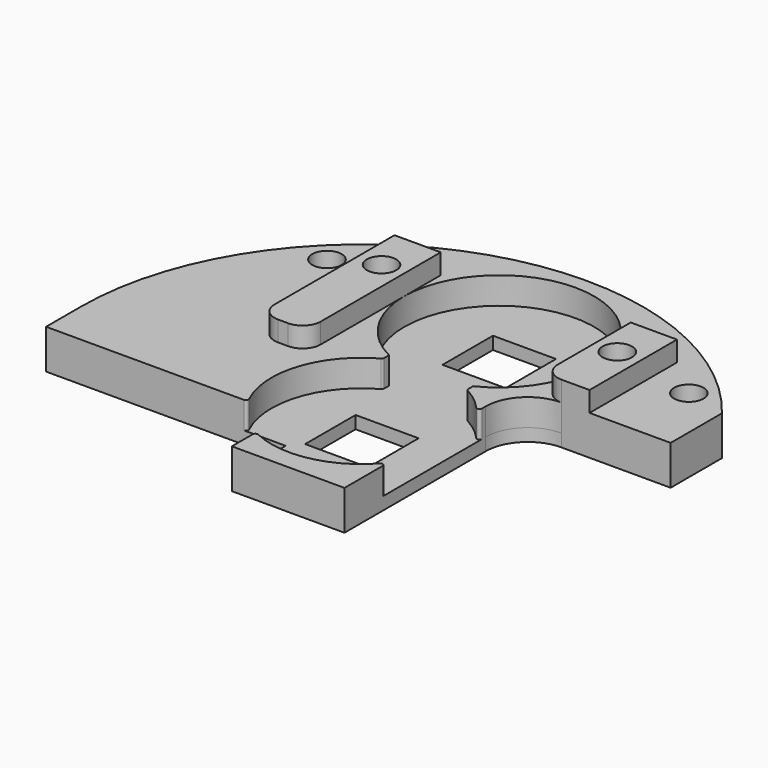
from build123d import *

# Parameters (mm, degrees)
F0_W      = 66.9
F0_H      = 51.6
F1_DEPTH  = 1.5
F2_R      = 33.44999
F3_R      = 1.75
F5_DEPTH  = 10
F6_W      = 60
F6_H      = 1.5
F7_DEPTH  = 7
F8_W      = 28.5
F8_H      = 1.5
F9_DEPTH  = 13
F10_W     = 18
F10_H     = 1.5
F11_DEPTH = 31
F12_R     = 5
F13_R     = 1.75
F13_R_2   = 11.3
F15_DEPTH = 3.2
F16_R     = 10.7
F17_DEPTH = 3.2
F18_W     = 10
F18_H     = 8
F19_DEPTH = 5
F14_W     = 7.5
F14_H     = 7.5
F20_DEPTH = 25
F21_W     = 13.4
F21_H     = 4.7
F22_DEPTH = 5
F23_W     = 5.5
F23_H     = 20
F23_H_2   = 13
F24_DEPTH = 2.4
F25_R     = 1.75
F26_DEPTH = 25
F27_R     = 2.15
F28_R     = 0.3


# Not quite as in the source:
# - a fillet or chamfer is up to 0.001 mm smaller than in the source, because OpenCascade refuses the exact size
# - ends of sketch curves that miss each other by under 0.0002 mm in the source are joined


with BuildPart() as f1:
    # F0 (on Top) → F1 (new body)
    with BuildSketch(Plane.XY):
        Rectangle(F0_W, F0_H)
    extrude(amount=F1_DEPTH)

    # F2 (radius 33.45 in the source; OpenCascade refuses exactly that, so slightly less here)
    f2_edges = [f1.edges().sort_by_distance(p)[0] for p in [
        (-33.45, 25.8, 0.75),
        (33.45, 25.8, 0.75),
    ]]
    fillet(f2_edges, radius=F2_R)

    # F3 (on Top) → F5 (cut)
    with BuildSketch(Plane.XY):
        with Locations((-21.525, 14.0641658831)):
            Circle(F3_R)
        with Locations((-14.025, 12.8033463032)):
            Circle(F3_R)
        with Locations((21.525, 14.0641658831)):
            Circle(F3_R)
        with Locations((14.025, 12.8033463032)):
            Circle(F3_R)
    extrude(amount=F5_DEPTH, mode=Mode.SUBTRACT)

    # F6 (on face) → F7 (cut)
    with BuildSketch(Plane.YZ.offset(33.45)):
        with Locations((4.2, 0.75)):
            Rectangle(F6_W, F6_H)
    extrude(amount=-F7_DEPTH, mode=Mode.SUBTRACT)

    # F8 (on face) → F9 (cut)
    with BuildSketch(Plane.XZ.offset(25.8)):
        with Locations((-19.2, 0.75)):
            Rectangle(F8_W, F8_H)
    extrude(amount=-F9_DEPTH, mode=Mode.SUBTRACT)

    # F10 (on face) → F11 (cut)
    with BuildSketch(Plane.XZ.offset(25.8)):
        with Locations((17.45, 0.75)):
            Rectangle(F10_W, F10_H)
    extrude(amount=-F11_DEPTH, mode=Mode.SUBTRACT)

    # F12
    f12_edges = [f1.edges().sort_by_distance(p)[0] for p in [
        (8.45, 5.2, 0.75),
    ]]
    fillet(f12_edges, radius=F12_R)

    # F13 (on face) → F15 (join)
    with BuildSketch(Plane.XY.offset(1.5)):
        with BuildLine():
            ThreePointArc((8.45, 0.2), (9.9144660941, 3.7355339059), (13.45, 5.2))
            Line((13.45, 5.2), (26.45, 5.2))
            Line((26.45, 5.2), (26.45, 12.8268227403))
            ThreePointArc((26.45, 12.8268227403), (14.7301262522, 22.3820846236), (1e-05, 25.8))
            ThreePointArc((1e-05, 25.8), (-23.6527247596, 16.0027247596), (-33.45, -7.64999))
            Line((-33.45, -7.64999), (-33.45, -12.8))
            Line((-33.45, -12.8), (-4.95, -12.8))
            Line((-4.95, -12.8), (-4.95, -25.8))
            Line((-4.95, -25.8), (8.45, -25.8))
            Line((8.45, -25.8), (8.45, 0.2))
        make_face()
        with Locations((-14.025, 12.8033463032)):
            Circle(F13_R, mode=Mode.SUBTRACT)
        with Locations((-21.525, 14.0641658831)):
            Circle(F13_R, mode=Mode.SUBTRACT)
        with Locations((0, 12.775)):
            Circle(F13_R_2, mode=Mode.SUBTRACT)
        with Locations((14.025, 12.8033463032)):
            Circle(F13_R, mode=Mode.SUBTRACT)
        with Locations((21.525, 14.0641658831)):
            Circle(F13_R, mode=Mode.SUBTRACT)
    extrude(amount=F15_DEPTH)

    # F16 (on face) → F17 (cut)
    with BuildSketch(Plane.XY.offset(1.5)):
        with Locations((0, -7.725)):
            Circle(F16_R)
    extrude(amount=F17_DEPTH, mode=Mode.SUBTRACT)

    # F18 (on face) → F19 (cut)
    with BuildSketch(Plane.XY.offset(1.5)):
        Rectangle(F18_W, F18_H)
    extrude(amount=F19_DEPTH, mode=Mode.SUBTRACT)

    # F14 (on face) → F20 (cut)
    with BuildSketch(Plane(origin=(0, 0, 0), x_dir=(1, 0, 0), z_dir=(0, 0, -1))):
        with Locations((0, -12.775)):
            Rectangle(F14_W, F14_H)
        with Locations((0, 7.65)):
            Rectangle(F14_W, F14_H)
    extrude(amount=-F20_DEPTH, mode=Mode.SUBTRACT)

    # F21 (on face) → F22 (cut)
    with BuildSketch(Plane.XZ.offset(25.8)):
        with Locations((1.75, 2.35)):
            Rectangle(F21_W, F21_H)
    extrude(amount=-F22_DEPTH, mode=Mode.SUBTRACT)

    # F23 (on face) → F24 (join)
    with BuildSketch(Plane.XY.offset(4.7)):
        with Locations((-14.05, 8.2)):
            Rectangle(F23_W, F23_H)
        with Locations((14.05, 11.7)):
            Rectangle(F23_W, F23_H_2)
    extrude(amount=F24_DEPTH)

    # F25 (on face) → F26 (cut)
    with BuildSketch(Plane(origin=(0, 0, 0), x_dir=(1, 0, 0), z_dir=(0, 0, -1))):
        with Locations((14.025, -12.8033463032)):
            Circle(F25_R)
        with Locations((-14.025, -12.8033463032)):
            Circle(F25_R)
    extrude(amount=-F26_DEPTH, mode=Mode.SUBTRACT)

    # F27
    f27_edges = [f1.edges().sort_by_distance(p)[0] for p in [
        (11.3, 5.2, 5.9),
        (-11.3, -1.8, 5.9),
        (-16.8, -1.8, 5.9),
    ]]
    fillet(f27_edges, radius=F27_R)

    # F28
    f28_edges = [f1.edges().sort_by_distance(p)[0] for p in [
        (-9.419893, -12.8, 3.1),
        (5, 1.734915, 3.1),
        (8.45, -1.160893, 3.1),
        (8.45, -14.289107, 3.1),
        (-4.95, -17.211174, 3.1),
        (-5, 1.734915, 3.1),
    ]]
    fillet(f28_edges, radius=F28_R)


solid = f1.part
